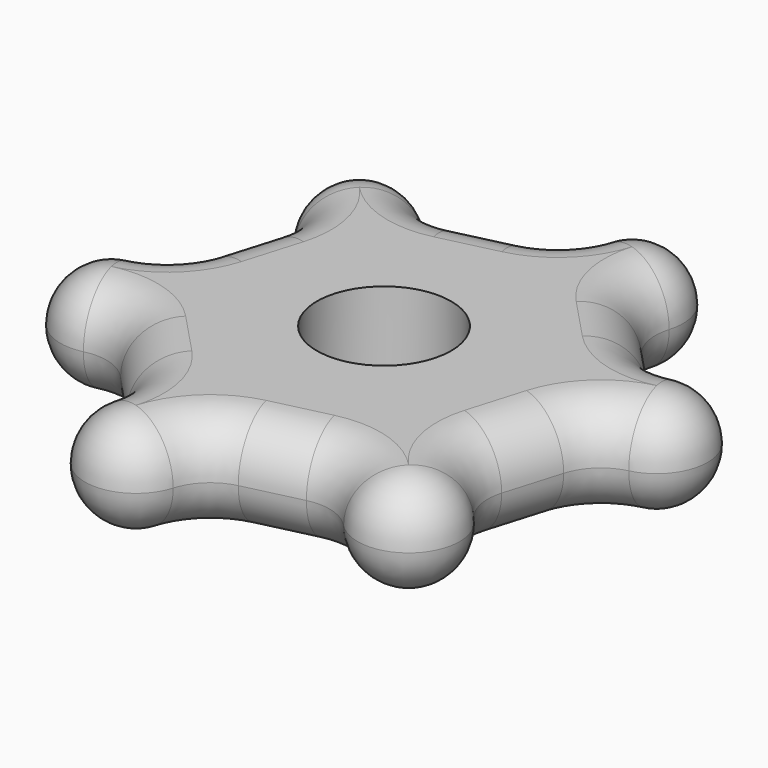
from build123d import *

# Parameters (mm, degrees)
F0_R     = 6.5804391212
F1_DEPTH = 10
F2_R     = 5
F3_R     = 4.99999


# Not quite as in the source:
# - a fillet or chamfer is up to 0.001 mm smaller than in the source, because OpenCascade refuses the exact size


with BuildPart() as f1:
    # F0 (on Top) → F1 (new body)
    with BuildSketch(Plane.XY):
        with BuildLine():
            Line((-1.8087860254, 20.1261428607), (-7.4263052889, 18.7931722466))
            ThreePointArc((-7.4263052889, 18.7931722466), (-10.0134209368, 18.8677539802), (-12.2166379436, 20.2259014802))
            ThreePointArc((-12.2166379436, 20.2259014802), (-19.2847693388, 20.4296625659), (-19.4885304245, 13.3615311707))
            ThreePointArc((-19.4885304245, 13.3615311707), (-18.2595622766, 11.0837324302), (-18.3341440102, 8.4966167823))
            Line((-18.3341440102, 8.4966167823), (-19.9885172277, 2.9652170869))
            ThreePointArc((-19.9885172277, 2.9652170869), (-21.3466647277, 0.7620000801), (-23.6244634681, -0.4669680679))
            ThreePointArc((-23.6244634681, -0.4669680679), (-27.3349914422, -6.4862688706), (-21.3156906395, -10.1967968447))
            ThreePointArc((-21.3156906395, -10.1967968447), (-18.7285749916, -10.2713785784), (-16.5253579848, -11.6295260784))
            Line((-16.5253579848, -11.6295260784), (-12.5622119388, -15.8279551597))
            ThreePointArc((-12.5622119388, -15.8279551597), (-11.3332437908, -18.1057539002), (-11.4078255245, -20.6928695481))
            ThreePointArc((-11.4078255245, -20.6928695481), (-8.0502221034, -26.9159314365), (-1.827160215, -23.5583280154))
            ThreePointArc((-1.827160215, -23.5583280154), (-0.469012715, -21.3551110086), (1.8087860254, -20.1261428607))
            Line((1.8087860254, -20.1261428607), (7.4263052889, -18.7931722466))
            ThreePointArc((7.4263052889, -18.7931722466), (10.0134209368, -18.8677539802), (12.2166379436, -20.2259014802))
            ThreePointArc((12.2166379436, -20.2259014802), (19.2847693388, -20.4296625659), (19.4885304245, -13.3615311707))
            ThreePointArc((19.4885304245, -13.3615311707), (18.2595622766, -11.0837324302), (18.3341440102, -8.4966167823))
            Line((18.3341440102, -8.4966167823), (19.9885172277, -2.9652170869))
            ThreePointArc((19.9885172277, -2.9652170869), (21.3466647277, -0.7620000801), (23.6244634681, 0.4669680679))
            ThreePointArc((23.6244634681, 0.4669680679), (27.3349914422, 6.4862688706), (21.3156906395, 10.1967968447))
            ThreePointArc((21.3156906395, 10.1967968447), (18.7285749916, 10.2713785784), (16.5253579848, 11.6295260784))
            Line((16.5253579848, 11.6295260784), (12.5622119388, 15.8279551597))
            ThreePointArc((12.5622119388, 15.8279551597), (11.3332437908, 18.1057539002), (11.4078255245, 20.6928695481))
            ThreePointArc((11.4078255245, 20.6928695481), (8.0502221034, 26.9159314365), (1.827160215, 23.5583280154))
            ThreePointArc((1.827160215, 23.5583280154), (0.469012715, 21.3551110086), (-1.8087860254, 20.1261428607))
        make_face()
        Circle(F0_R, mode=Mode.SUBTRACT)
    extrude(amount=F1_DEPTH)

    # F2
    f2_edges = [f1.edges().sort_by_distance(p)[0] for p in [
        (-19.284769, 20.429663, 10),
        (-10.013421, 18.867754, 10),
        (-4.617546, 19.459658, 10),
    ]]
    fillet(f2_edges, radius=F2_R)

    # F3 (radius 5 in the source; OpenCascade refuses exactly that, so slightly less here)
    f3_edges = [f1.edges().sort_by_distance(p)[0] for p in [
        (-27.334991, -6.486269, 0),
    ]]
    fillet(f3_edges, radius=F3_R)


solid = f1.part
